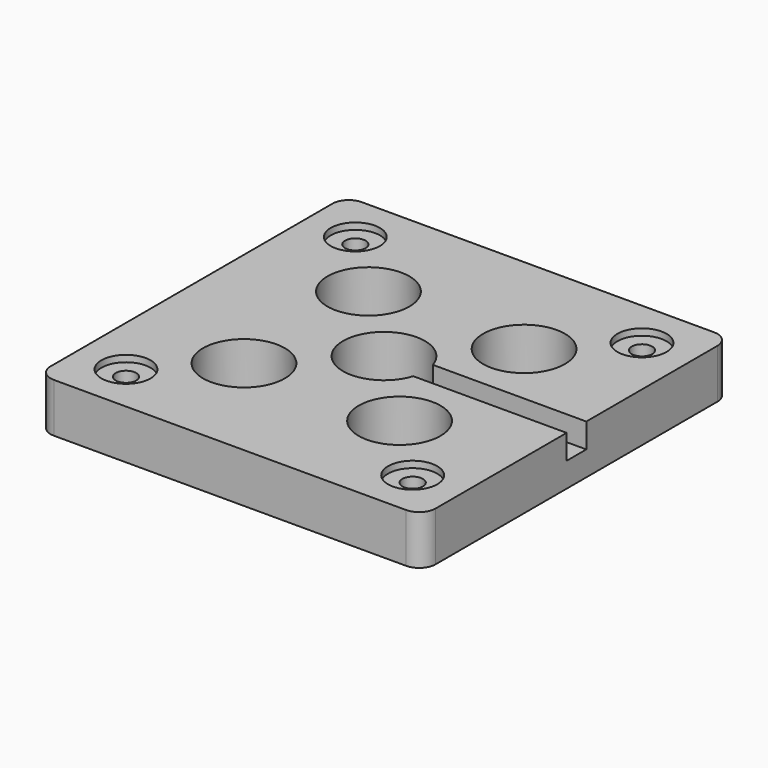
from build123d import *

# Parameters (mm, degrees)
F0_R     = 3.9751
F0_R_2   = 15.875
F0_R_3   = 3.96875
F1_DEPTH = 19.05
F3_DEPTH = 9.525
F5_R     = 9.525
F5_R_2   = 3.9751
F5_R_3   = 3.96875
F6_DEPTH = 2.54


# Not quite as in the source:
# - a feature of the source that left no trace in its solid (it failed there, or was rolled back) is left out


with BuildPart() as f1:
    # F0 (on Top) → F1 (new body)
    with BuildSketch(Plane.XY):
        with BuildLine():
            Line((-68.2625, -74.6125), (68.2625, -74.6125))
            ThreePointArc((68.2625, -74.6125), (72.7526280605, -72.7526280605), (74.6125, -68.2625))
            Line((74.6125, -68.2625), (74.6125, -4.7625))
            Line((74.6125, -4.7625), (15.1437848225, -4.7625))
            ThreePointArc((15.1437848225, -4.7625), (-15.875, 0), (15.1437848225, 4.7625))
            Line((15.1437848225, 4.7625), (74.6125, 4.7625))
            Line((74.6125, 4.7625), (74.6125, 68.2625))
            ThreePointArc((74.6125, 68.2625), (72.7526280605, 72.7526280605), (68.2625, 74.6125))
            Line((68.2625, 74.6125), (-68.2625, 74.6125))
            ThreePointArc((-68.2625, 74.6125), (-72.7526280605, 72.7526280605), (-74.6125, 68.2625))
            Line((-74.6125, 68.2625), (-74.6125, -68.2625))
            ThreePointArc((-74.6125, -68.2625), (-72.7526280605, -72.7526280605), (-68.2625, -74.6125))
        make_face()
        with Locations((-55.5625, -55.5625)):
            Circle(F0_R, mode=Mode.SUBTRACT)
        with Locations((-30.1625, -30.1625)):
            Circle(F0_R_2, mode=Mode.SUBTRACT)
        with Locations((55.5625, -55.5625)):
            Circle(F0_R, mode=Mode.SUBTRACT)
        with Locations((30.1625, -30.1625)):
            Circle(F0_R_2, mode=Mode.SUBTRACT)
        with Locations((-30.1625, 30.1625)):
            Circle(F0_R_2, mode=Mode.SUBTRACT)
        with Locations((-55.5625, 55.5625)):
            Circle(F0_R_3, mode=Mode.SUBTRACT)
        with Locations((30.1625, 30.1625)):
            Circle(F0_R_2, mode=Mode.SUBTRACT)
        with Locations((55.5625, 55.5625)):
            Circle(F0_R, mode=Mode.SUBTRACT)
    extrude(amount=F1_DEPTH)

    # F2 (on face) → F3 (join)
    with BuildSketch(Plane(origin=(0, 0, 0), x_dir=(1, 0, 0), z_dir=(0, 0, -1))):
        with BuildLine():
            Line((74.6125, 4.7625), (15.1437848225, 4.7625))
            ThreePointArc((15.1437848225, 4.7625), (15.875, 0), (15.1437848225, -4.7625))
            Line((15.1437848225, -4.7625), (74.6125, -4.7625))
            Line((74.6125, -4.7625), (74.6125, 4.7625))
        make_face()
    extrude(amount=-F3_DEPTH)

    # F5 (on face) → F6 (cut)
    with BuildSketch(Plane.XY.offset(19.05)):
        with Locations((-55.5625, -55.5625)):
            Circle(F5_R)
        with Locations((-55.5625, -55.5625)):
            Circle(F5_R_2, mode=Mode.SUBTRACT)
        with Locations((55.5625, -55.5625)):
            Circle(F5_R)
        with Locations((55.5625, -55.5625)):
            Circle(F5_R_2, mode=Mode.SUBTRACT)
        with Locations((55.5625, 55.5625)):
            Circle(F5_R)
        with Locations((55.5625, 55.5625)):
            Circle(F5_R_2, mode=Mode.SUBTRACT)
        with Locations((-55.5625, 55.5625)):
            Circle(F5_R)
        with Locations((-55.5625, 55.5625)):
            Circle(F5_R_3, mode=Mode.SUBTRACT)
    extrude(amount=-F6_DEPTH, mode=Mode.SUBTRACT)


solid = f1.part
